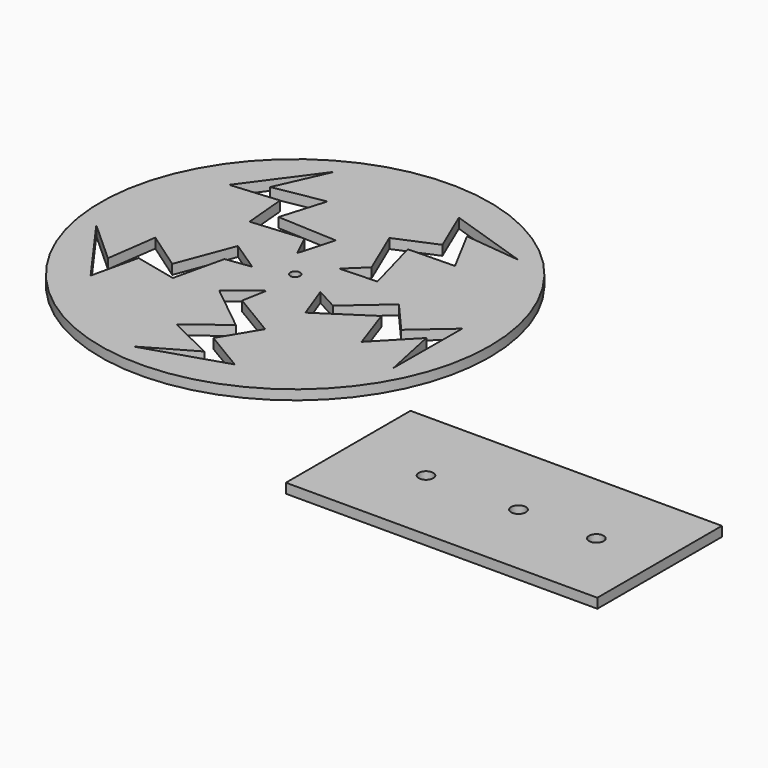
from build123d import *

# Parameters (mm, degrees)
F0_W     = 101.6
F0_H     = 50.8
F1_DEPTH = 3.175
F3_DEPTH = 3.176
F5_R     = 63.5
F5_R_2   = 1.5875
F6_DEPTH = 3.175


# Not quite as in the source:
# - a length typed as a fraction of an inch, garbled in the dataset ("3 / 203.2 mm" for 3/8 in), is restored


with BuildPart() as f1:
    # F0 (on Top) → F1 (new body)
    with BuildSketch(Plane.XY):
        with Locations((50.8, -25.4)):
            Rectangle(F0_W, F0_H)
    extrude(amount=F1_DEPTH)

    # F2 (on face) → F3 (cut, through all)
    with BuildSketch(Plane.XY.offset(3.175)):
        with BuildLine():
            ThreePointArc((27.78125, -25.4), (25.4, -23.01875), (23.01875, -25.4))
            Line((23.01875, -25.4), (25.4, -25.4))
            Line((25.4, -25.4), (27.78125, -25.4))
        make_face()
        with BuildLine():
            Line((25.4, -25.4), (23.01875, -25.4))
            ThreePointArc((23.01875, -25.4), (25.4, -27.78125), (27.78125, -25.4))
            Line((27.78125, -25.4), (25.4, -25.4))
        make_face()
        with BuildLine():
            Line((55.5625, -25.4), (53.1749, -25.4))
            ThreePointArc((53.1749, -25.4), (55.5625, -27.7876), (57.9501, -25.4))
            Line((57.9501, -25.4), (55.5625, -25.4))
        make_face()
        with BuildLine():
            ThreePointArc((57.9501, -25.4), (55.5625, -23.0124), (53.1749, -25.4))
            Line((53.1749, -25.4), (55.5625, -25.4))
            Line((55.5625, -25.4), (57.9501, -25.4))
        make_face()
        with BuildLine():
            ThreePointArc((83.3501, -25.4), (80.9625, -23.0124), (78.5749, -25.4))
            ThreePointArc((78.5749, -25.4), (80.9625, -27.7876), (83.3501, -25.4))
        make_face()
    extrude(amount=-F3_DEPTH, mode=Mode.SUBTRACT)


with BuildPart() as f6:
    # F5 (on Top) → F6 (new body)
    with BuildSketch(Plane.XY):
        with Locations((-69.9992328882, 40.4729917645)):
            Circle(F5_R)
        Polygon((-91.1287275403, 43.5456714677), (-81.1082634294, 36.8634489357), (-89.266684788, 35.7642112787), (-93.0278924051, 19.3807095608), (-106.7233378314, 22.5248123628), (-110.209272308, 7.3403771227), (-126.4287452471, 29.9333454927), (-112.7548140407, 17.5712748797), (-110.4600478416, 34.0252232445), (-98.0220682083, 25.3789987215), align=None, mode=Mode.SUBTRACT)
        Polygon((-79.4508978724, 21.3271584362), (-69.9992328882, 28.7922658026), (-71.4748865987, 20.6934628899), (-57.0555276033, 12.0535614183), (-64.2778724432, 0), (-50.9138293564, -8.0075692385), (-77.4131119251, -16.4515934885), (-61.4306069911, -7.2670020163), (-76.3701200485, 0), (-64.3035247922, 9.157391265), align=None, mode=Mode.SUBTRACT)
        Polygon((-54.7111884466, 25.5675363215), (-58.8902023471, 36.8634489357), (-51.6437851371, 32.9573511244), (-38.9709235648, 44.0011000734), (-29.7391327281, 33.4074866294), (-17.9937653968, 43.6429719128), (-18.1517497626, 15.8313095546), (-21.9479496944, 33.8697698701), (-33.4758427384, 21.9070757477), (-38.4562563748, 36.2128793208), align=None, mode=Mode.SUBTRACT)
        Polygon((-73.6063137641, 61.517845586), (-76.8649913447, 49.9228975744), (-80.4315193284, 57.3423342534), (-97.17543247, 55.8566748086), (-98.4173383945, 69.8533986226), (-113.9358074704, 68.4764707828), (-97.4607104577, 90.8837173921), (-104.9922611464, 74.0589461098), (-88.6345045816, 76.9610434321), (-93.0140056732, 62.4599915375), align=None, mode=Mode.SUBTRACT)
        with Locations((-69.9992328882, 40.4729917645)):
            Circle(F5_R_2, mode=Mode.SUBTRACT)
        Polygon((-51.0990368176, 50.4067470113), (-63.1334744317, 49.9228975744), (-57.1792885888, 55.6075992763), (-63.7663883979, 71.0729129616), (-50.8384830438, 76.5792612079), (-56.9434899095, 90.9127082429), (-30.5418470485, 82.1681798718), (-48.8705325686, 84.1319699794), (-41.0556492309, 69.4716163984), (-56.2003093926, 69.1556979779), align=None, mode=Mode.SUBTRACT)
    extrude(amount=F6_DEPTH)


solid = Compound([f1.part, f6.part])
